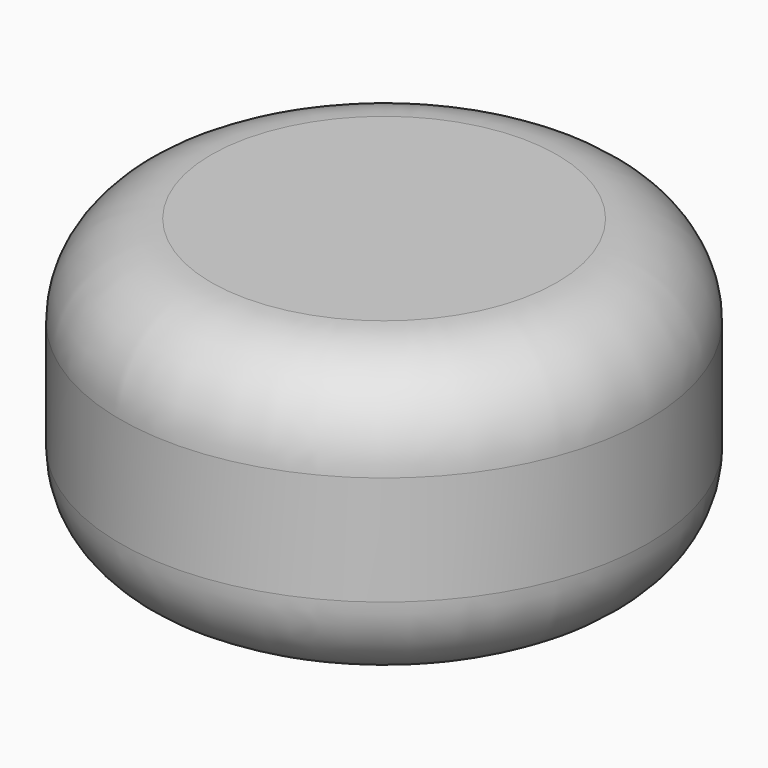
from build123d import *

# Parameters (mm, degrees)
F1_R     = 14.5
F2_DEPTH = 8
F4_DEPTH = 5.5
F5_R     = 5


with BuildPart() as f2:
    # F1 (on Top) → F2 (new body, symmetric)
    with BuildSketch(Plane.XY):
        Circle(F1_R)
    extrude(amount=F2_DEPTH, both=True)

    # F3 (on Top) → F4 (cut, symmetric)
    with BuildSketch(Plane.XY):
        Polygon((-11.1578674376, 0), (-5.6730398803, -9.5), (5.2966152343, -9.5), (10.7814427916, 0), (5.2966152343, 9.5), (-5.6730398803, 9.5), align=None)
    extrude(amount=F4_DEPTH, both=True, mode=Mode.SUBTRACT)

    # F5
    f5_edges = [f2.edges().sort_by_distance(p)[0] for p in [
        (-14.5, 0, 8),
        (-14.5, 0, -8),
    ]]
    fillet(f5_edges, radius=F5_R)


solid = f2.part
